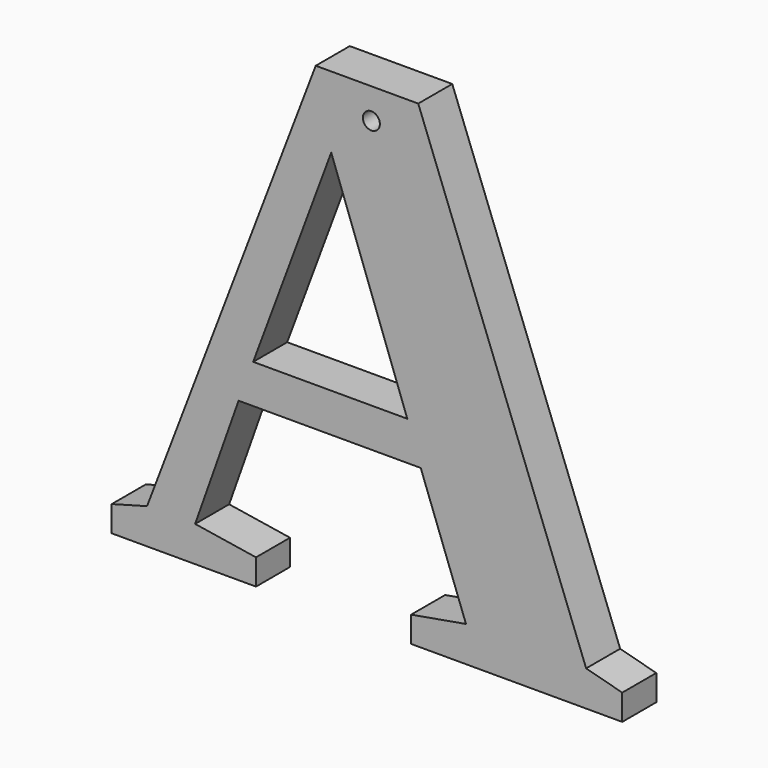
from build123d import *

# Parameters (mm, degrees)
F0_TEXT_SIZE = 108.1213303324
F2_DEPTH     = 6.35
F3_D         = 2.54


# Not quite as in the source:
# - Text() gives the source's letters only with a copy of the font that has no kerning and outlines rounded to 1/6400 em; it was checked with that copy


with BuildPart() as f2:
    # F0 (on Front) → F2 (new body)
    with BuildSketch(Plane.XZ):
        with Locations((-56.6064678133, -39.9333760142)):
            Text('A', F0_TEXT_SIZE, font='Tinos', font_style=FontStyle.BOLD, text_align=(TextAlign.LEFT, TextAlign.BOTTOM))
    extrude(amount=F2_DEPTH)

    # F3 (through all)
    with Locations(Plane(origin=(0, 0, 0), x_dir=(1, 0, 0), z_dir=(0, 1, 0))):
        with Locations((-16.776939854, -26.8966499716)):
            Hole(F3_D / 2)


solid = f2.part
